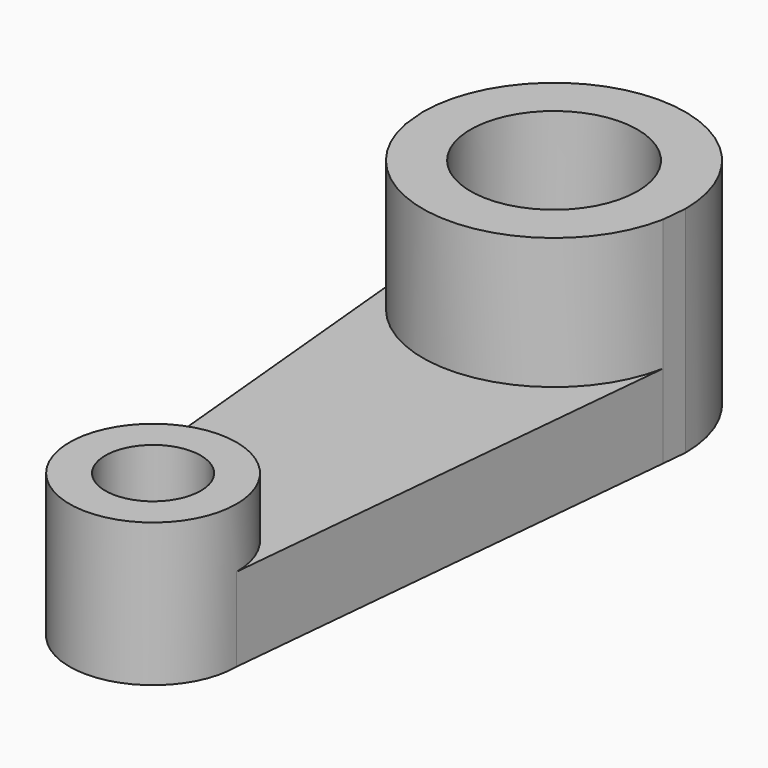
from build123d import *

# Parameters (mm, degrees)
F0_R     = 22.225
F0_R_2   = 12.7
F1_DEPTH = 22.225
F2_R     = 22.225
F3_DEPTH = 34.925
F4_DEPTH = 50.8
F5_R     = 12.7
F6_DEPTH = 15.875
F7_R     = 12.7
F8_DEPTH = 38.1


# Not quite as in the source:
# - a length typed as a fraction of an inch, garbled in the dataset ("3 / 203.2 mm" for 3/8 in), is restored


with BuildPart() as f1:
    # F0 (on Top) → F1 (new body)
    with BuildSketch(Plane.XY):
        with BuildLine():
            Line((22.225, 0), (34.2971348315, 126.7574157303))
            ThreePointArc((34.2971348315, 126.7574157303), (0, 98.425), (-34.2971348315, 126.7574157303))
            Line((-34.2971348315, 126.7574157303), (-22.225, 0))
            ThreePointArc((-22.225, 0), (0, 22.225), (22.225, 0))
        make_face()
        with BuildLine():
            Line((34.2971348315, 126.7574157303), (34.925, 133.35))
            ThreePointArc((34.925, 133.35), (0, 168.275), (-34.925, 133.35))
            Line((-34.925, 133.35), (-34.2971348315, 126.7574157303))
            ThreePointArc((-34.2971348315, 126.7574157303), (0, 98.425), (34.2971348315, 126.7574157303))
        make_face()
        with Locations((0, 133.35)):
            Circle(F0_R, mode=Mode.SUBTRACT)
        with BuildLine():
            ThreePointArc((-22.225, 0), (0, -22.225), (22.225, 0))
            ThreePointArc((22.225, 0), (0, 22.225), (-22.225, 0))
        make_face()
        Circle(F0_R_2, mode=Mode.SUBTRACT)
        with Locations((0, 133.35)):
            Circle(F0_R)
        Circle(F0_R_2)
    extrude(amount=F1_DEPTH)

    # F2 (on face) → F3 (join)
    with BuildSketch(Plane.XY.offset(22.225)):
        with BuildLine():
            ThreePointArc((-34.2971348315, 126.7574157303), (0, 98.425), (34.2971348315, 126.7574157303))
            Line((34.2971348315, 126.7574157303), (34.925, 133.35))
            ThreePointArc((34.925, 133.35), (0, 168.275), (-34.925, 133.35))
            Line((-34.925, 133.35), (-34.2971348315, 126.7574157303))
        make_face()
        with Locations((0, 133.35)):
            Circle(F2_R, mode=Mode.SUBTRACT)
    extrude(amount=F3_DEPTH)

    # F4 (cut): a face of the model
    f4_faces = [f1.faces().sort_by_distance(p)[0] for p in [
        (0, 133.35, 22.225),
    ]]
    extrude(f4_faces, amount=-F4_DEPTH, mode=Mode.SUBTRACT)

    # F5 (on face) → F6 (join)
    with BuildSketch(Plane.XY.offset(22.225)):
        with BuildLine():
            ThreePointArc((-22.225, 0), (0, -22.225), (22.225, 0))
            ThreePointArc((22.225, 0), (0, 22.225), (-22.225, 0))
        make_face()
        Circle(F5_R, mode=Mode.SUBTRACT)
        Circle(F5_R)
    extrude(amount=F6_DEPTH)

    # F7 (on face) → F8 (cut)
    with BuildSketch(Plane.XY.offset(38.1)):
        Circle(F7_R)
    extrude(amount=-F8_DEPTH, mode=Mode.SUBTRACT)


solid = f1.part
